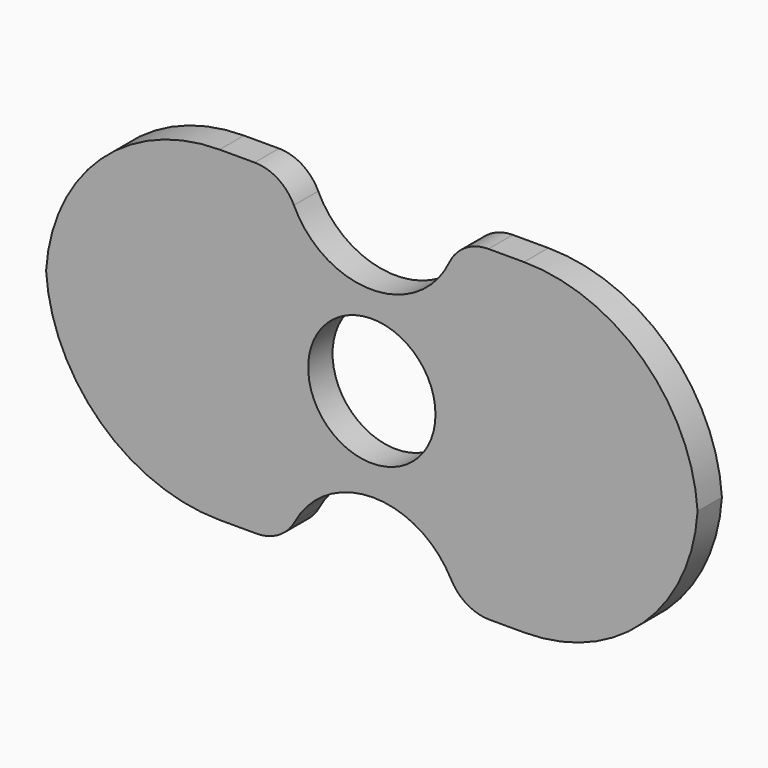
from build123d import *

# Parameters (mm, degrees)
F0_R        = 3.7178453792
F1_DEPTH    = 0.889
F2_T1_DEPTH = 52.578
F3_R        = 2.54


# Not quite as in the source:
# - a fillet or chamfer that OpenCascade refuses, or shapes differently, is made with other operations: its cross-section is extruded or revolved along the edge and cut away or added


with BuildPart() as f1:
    # F0 (on Front) → F1 (new body, symmetric)
    with BuildSketch(Plane.XZ):
        with BuildLine():
            Line((19.05, -9.525), (19.05, 9.525))
            Line((19.05, 9.525), (4.9566612579, 9.525))
            ThreePointArc((4.9566612579, 9.525), (-0.016463222, 5.2090361219), (-4.9895877019, 9.525))
            Line((-4.9895877019, 9.525), (-19.05, 9.525))
            Line((-19.05, 9.525), (-19.05, -9.525))
            Line((-19.05, -9.525), (-4.9895877019, -9.525))
            ThreePointArc((-4.9895877019, -9.525), (0.067827059, -5.4479951467), (5.1252418198, -9.525))
            Line((5.1252418198, -9.525), (19.05, -9.525))
        make_face()
        Circle(F0_R, mode=Mode.SUBTRACT)
    extrude(amount=F1_DEPTH, both=True)

    # F2: fillet of radius 10.16 on 4 edges, made by hand

    # F2_s2 → F2_t1 (cut)
    with BuildSketch(Plane.XZ.offset(-26.289)):
        with BuildLine():
            ThreePointArc((-19.05, -0.635), (-16.0742048969, 6.5492048969), (-8.89, 9.525))
            Line((-8.89, 9.525), (-19.05, 9.525))
            Line((-19.05, 9.525), (-19.05, -0.635))
        make_face()
        with BuildLine():
            ThreePointArc((-8.89, -9.525), (-16.0742048969, -6.5492048969), (-19.05, 0.635))
            Line((-19.05, 0.635), (-19.05, -9.525))
            Line((-19.05, -9.525), (-8.89, -9.525))
        make_face()
        with BuildLine():
            ThreePointArc((8.89, 9.525), (16.0742048969, 6.5492048969), (19.05, -0.635))
            Line((19.05, -0.635), (19.05, 9.525))
            Line((19.05, 9.525), (8.89, 9.525))
        make_face()
        with BuildLine():
            ThreePointArc((19.05, 0.635), (16.0742048969, -6.5492048969), (8.89, -9.525))
            Line((8.89, -9.525), (19.05, -9.525))
            Line((19.05, -9.525), (19.05, 0.635))
        make_face()
    extrude(amount=F2_T1_DEPTH, mode=Mode.SUBTRACT)

    # F3
    f3_edges = [f1.edges().sort_by_distance(p)[0] for p in [
        (-4.989588, 0, 9.525),
        (5.125242, 0, -9.525),
        (-4.989588, 0, -9.525),
        (4.956661, 0, 9.525),
    ]]
    fillet(f3_edges, radius=F3_R)


solid = f1.part
